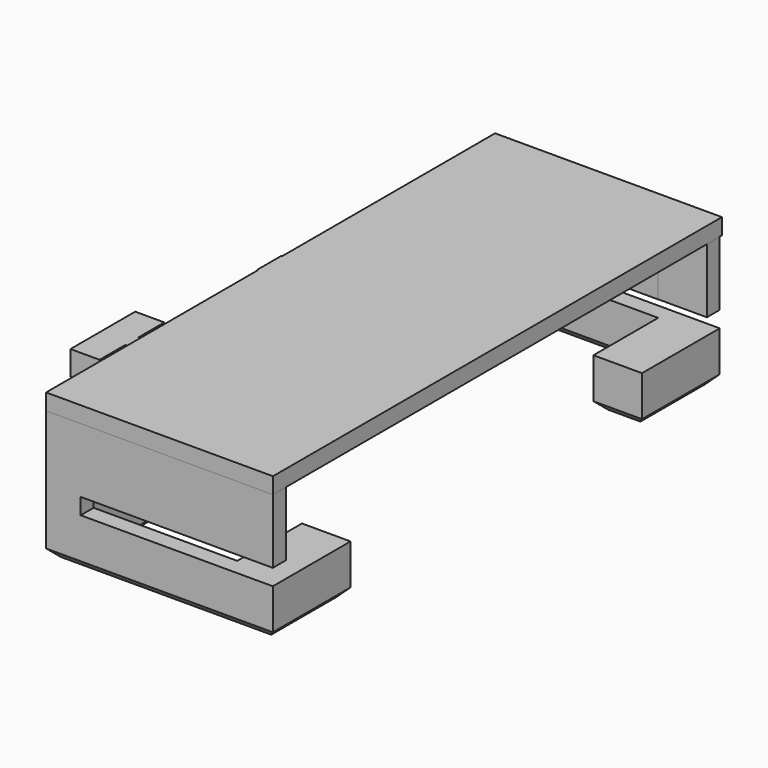
from build123d import *

# Parameters (mm, degrees)
F1_DEPTH  = 18
F2_SIZE   = 0.99999
F4_W      = 49.3712280877
F4_H      = 16.5352197364
F6_W      = 25.0472677872
F6_H      = 14.5927555859
F8_W      = 28.0247684568
F8_H      = 69.3199932575
F9_DEPTH  = 2
F11_W     = 7.2507392615
F11_H     = 64.9974308908
F12_DEPTH = 10
F13_W     = 37.7304842696
F13_H     = 75.3901228309
F14_DEPTH = 2


# Not quite as in the source:
# - a fillet or chamfer is up to 0.001 mm smaller than in the source, because OpenCascade refuses the exact size


with BuildPart() as f1:
    # F0 (on Top) → F1 (new body)
    with BuildSketch(Plane.XY):
        Polygon((-8.5048572017, 5), (-12.1048572017, 5), (-12.1048572017, 0), (-12.1048572017, -5), (-8.5048572017, -5), (-8.5048572017, -1), (6.4951427983, -1), (8.4951427983, -3.4849380649), (8.4951427983, -34.5), (36.4951427983, -34.5), (36.4951427983, -22.5), (30.4951427983, -22.5), (30.4951427983, -32.5), (12.4951427983, -32.5), (12.4951427983, 0), (12.4951427983, 32.5), (30.4951427983, 32.5), (30.4951427983, 22.5), (36.4951427983, 22.5), (36.4951427983, 34.5), (8.4951427983, 34.5), (8.4951427983, 3.4849380649), (6.4951427983, 1), (-8.5048572017, 1), align=None)
    extrude(amount=F1_DEPTH)

    # F2 (size 1 in the source; OpenCascade refuses exactly that, so slightly less here)
    f2_edges = [f1.edges().sort_by_distance(p)[0] for p in [
        (-10.304857, 5, 18),
        (-12.104857, 0, 18),
        (-10.304857, -5, 18),
        (-8.504857, -3, 18),
        (-1.004857, -1, 18),
        (7.495143, -2.242469, 18),
        (8.495143, -18.992469, 18),
        (22.495143, -34.5, 18),
        (36.495143, -28.5, 18),
        (33.495143, -22.5, 18),
        (30.495143, -27.5, 18),
        (21.495143, -32.5, 18),
        (12.495143, 0, 18),
        (21.495143, 32.5, 18),
        (30.495143, 27.5, 18),
        (33.495143, 22.5, 18),
        (36.495143, 28.5, 18),
        (22.495143, 34.5, 18),
        (8.495143, 18.992469, 18),
        (7.495143, 2.242469, 18),
        (-1.004857, 1, 18),
        (-8.504857, 3, 18),
        (-10.304857, 5, 0),
        (-12.104857, 0, 0),
        (-10.304857, -5, 0),
        (-8.504857, -3, 0),
        (-1.004857, -1, 0),
        (7.495143, -2.242469, 0),
        (8.495143, -18.992469, 0),
        (22.495143, -34.5, 0),
        (36.495143, -28.5, 0),
        (33.495143, -22.5, 0),
        (30.495143, -27.5, 0),
        (21.495143, -32.5, 0),
        (12.495143, 0, 0),
        (21.495143, 32.5, 0),
        (30.495143, 27.5, 0),
        (33.495143, 22.5, 0),
        (36.495143, 28.5, 0),
        (22.495143, 34.5, 0),
        (8.495143, 18.992469, 0),
        (7.495143, 2.242469, 0),
        (-1.004857, 1, 0),
        (-8.504857, 3, 0),
    ]]
    chamfer(f2_edges, length=F2_SIZE)

    # F4 (on offset) → F7 section 0
    with BuildSketch(Plane.XY.offset(4)):
        with Locations((-18.2442103978, -0.0910270028)):
            Rectangle(F4_W, F4_H)
    # F6 (on offset) → F7 section 1
    with BuildSketch(Plane.XY.offset(18)):
        with Locations((-4.1036796756, 0.1169494353)):
            Rectangle(F6_W, F6_H)
    loft(mode=Mode.SUBTRACT)

    # F8 (on offset) → F9 (join)
    with BuildSketch(Plane.XY.offset(18)):
        with Locations((22.5351126865, 0.1127310097)):
            Rectangle(F8_W, F8_H)
    extrude(amount=-F9_DEPTH)

    # F11 (on offset) → F12 (cut)
    with BuildSketch(Plane.XY.offset(6)):
        with Locations((34.090702422, 0.0231582671)):
            Rectangle(F11_W, F11_H)
    extrude(amount=F12_DEPTH, mode=Mode.SUBTRACT)

    # F13 (on offset) → F14 (cut)
    with BuildSketch(Plane.XY.offset(6)):
        with Locations((31.6290971823, -0.1884736121)):
            Rectangle(F13_W, F13_H)
    extrude(amount=F14_DEPTH, mode=Mode.SUBTRACT)


solid = f1.part
